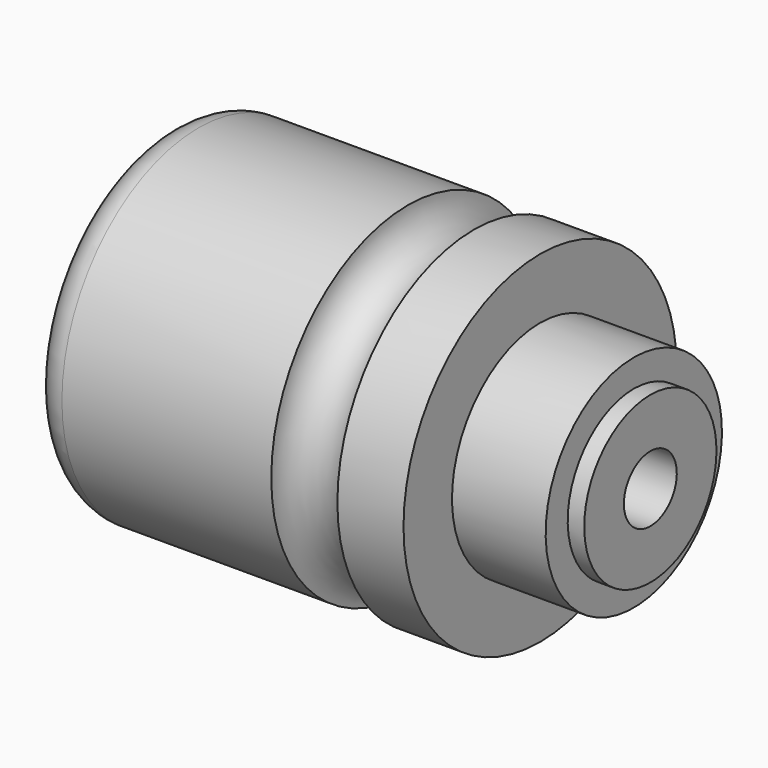
from build123d import *

# Parameters (mm, degrees)
F4_R = 5.99999


# Not quite as in the source:
# - a fillet or chamfer is up to 0.001 mm smaller than in the source, because OpenCascade refuses the exact size


with BuildPart() as f1:
    # F0 (on Front) → F1 (revolve)
    with BuildSketch(Plane.XZ):
        with BuildLine():
            Line((0, 31), (0, 0))
            Line((0, 0), (88, 0))
            Line((88, 0), (88, 15))
            Line((88, 15), (85, 15))
            Line((85, 15), (85, 20))
            Line((85, 20), (68, 20))
            Line((68, 20), (68, 31))
            Line((68, 31), (56, 31))
            ThreePointArc((56, 31), (50, 25), (44, 31))
            Line((44, 31), (0, 31))
        make_face()
    revolve(axis=Axis((48.1394192929, 0, 0), (1, 0, 0)))

    # F2 (on Front) → F3 (revolve, cut)
    with BuildSketch(Plane.XZ):
        Polygon((0, 25), (0, 0), (88, 0), (88, 6), (30, 6), (30, 16), (22, 16), (22, 20.5), (15, 20.5), (15, 12.5), (12, 12.5), (12, 16), (1.5, 16), (1.5, 25), align=None)
    revolve(axis=Axis((-13.0126860076, 0, 0), (-1, 0, 0)), mode=Mode.SUBTRACT)

    # F4 (radius 6 in the source; OpenCascade refuses exactly that, so slightly less here)
    f4_edges = [f1.edges().sort_by_distance(p)[0] for p in [
        (0, 0, -31),
    ]]
    fillet(f4_edges, radius=F4_R)


solid = f1.part
